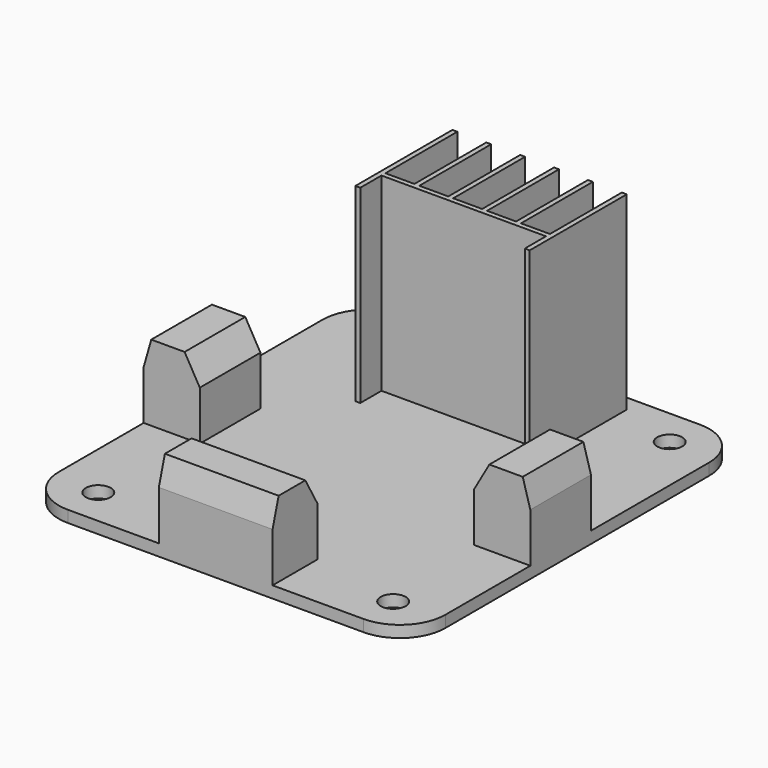
from build123d import *

# Parameters (mm, degrees)
F1_DEPTH  = 1.54
F3_D      = 3.3
F5_DEPTH  = 25
F8_DEPTH  = 10
F10_DEPTH = 7.5


# Not quite as in the source:
# - a pattern or mirror of a feature is missing from the dataset's text; its kind, count and spacing are read off the source's solid


with BuildPart() as f1:
    # F0 (on Top) → F1 (new body)
    with BuildSketch(Plane.XY):
        with BuildLine():
            Line((-19.5, -27.75), (19.5, -27.75))
            ThreePointArc((19.5, -27.75), (23.7426406871, -25.9926406871), (25.5, -21.75))
            Line((25.5, -21.75), (25.5, 21.75))
            ThreePointArc((25.5, 21.75), (23.7426406871, 25.9926406871), (19.5, 27.75))
            Line((19.5, 27.75), (-19.5, 27.75))
            ThreePointArc((-19.5, 27.75), (-23.7426406871, 25.9926406871), (-25.5, 21.75))
            Line((-25.5, 21.75), (-25.5, -21.75))
            ThreePointArc((-25.5, -21.75), (-23.7426406871, -25.9926406871), (-19.5, -27.75))
        make_face()
    extrude(amount=F1_DEPTH)

    # F3 (through all)
    with Locations(Plane.XY.offset(1.54)):
        with Locations((-19.45, 22.8), (19.45, 22.8), (-19.45, -22.8), (19.45, -22.8)):
            Hole(F3_D / 2)

    # F4 (on face) → F5 (join)
    with BuildSketch(Plane.XY.offset(1.54)):
        Polygon((10.85, 9.65), (11.5, 9.65), (11.5, 25.65), (10.85, 25.65), (10.85, 13.7976789847), (7.03, 13.7976789847), (7.03, 25.65), (6.38, 25.65), (6.38, 13.7976789847), (2.56, 13.7976789847), (2.56, 25.65), (1.91, 25.65), (1.91, 13.7976789847), (-1.91, 13.7976789847), (-1.91, 25.65), (-2.56, 25.65), (-2.56, 13.7976789847), (-6.38, 13.7976789847), (-6.38, 25.65), (-7.03, 25.65), (-7.03, 13.7976789847), (-10.85, 13.7976789847), (-10.85, 25.65), (-11.5, 25.65), (-11.5, 9.65), (-10.85, 9.65), (-10.85, 13.1476789847), (10.85, 13.1476789847), align=None)
    extrude(amount=F5_DEPTH)

    # F7 (on offset) → F8 (join)
    with BuildSketch(Plane.XZ.offset(7.75)):
        Polygon((18.1, 1.54), (25.5, 1.54), (25.5, 8.04), (24.5, 11.54), (20.1, 11.54), (18.1, 8.04), align=None)
    f8 = extrude(amount=-F8_DEPTH)

    # F8_copies: F8 across plane
    add(f8.mirror(Plane(origin=(0, 0, 0), x_dir=(0, 0, -1), z_dir=(-1, 0, 0))))

    # F9 (on Right) → F10 (join, symmetric)
    with BuildSketch(Plane.YZ):
        Polygon((-27.75, 1.54), (-20.35, 1.54), (-20.35, 8.04), (-22.35, 11.54), (-26.75, 11.54), (-27.75, 8.04), align=None)
    extrude(amount=F10_DEPTH, both=True)


solid = f1.part
